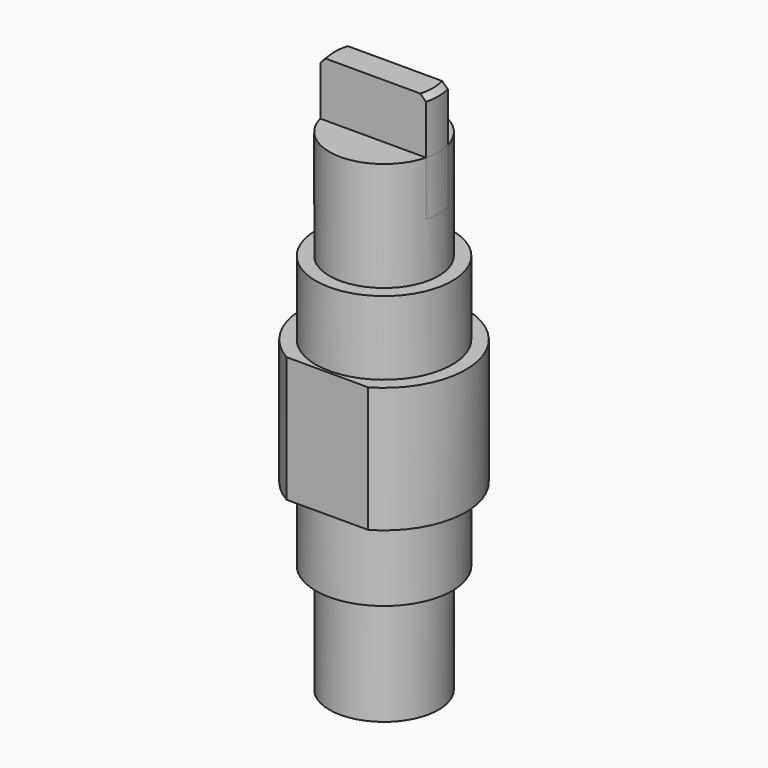
from build123d import *
from build123d import SkipClean  # not in build123d's __all__

# Parameters (mm, degrees)
F3_DEPTH      = 25
F3_DEPTH_BACK = 25
F6_DEPTH      = 10
F6_DEPTH_BACK = 10
F7_SIZE       = 1


with BuildPart() as f1:
    # F0 (on Front) → F1 (revolve)
    with BuildSketch(Plane.XZ):
        Polygon((-12.5, 11.5), (-15, 11.5), (-15, 0), (-15, -11.5), (-12.5, -11.5), (-12.5, -25), (-10, -25), (-10, -45), (0, -45), (0, 0), (0, 45), (-10, 45), (-10, 25), (-12.5, 25), align=None)
    revolve(axis=Axis((0, 0, 22.5), (0, 0, -1)))

    # F2 (on Top) → F3 (cut, two sides)
    with BuildSketch(Plane.XY) as f3_sk:
        Polygon((0, -13), (-15, -13), (-15, -17), (0, -17), (15, -17), (15, -13), align=None)
    extrude(amount=F3_DEPTH, mode=Mode.SUBTRACT)
    extrude(f3_sk.sketch, amount=-F3_DEPTH_BACK, mode=Mode.SUBTRACT)

    # F5 (on offset) → F6 (join, two sides)
    with BuildSketch(Plane.XY.offset(45)) as f6_sk:
        with BuildLine():
            Line((9.6824583655, 2.5), (-9.6824583655, 2.5))
            ThreePointArc((-9.6824583655, 2.5), (-10, 0), (-9.6824583655, -2.5))
            Line((-9.6824583655, -2.5), (9.6824583655, -2.5))
            ThreePointArc((9.6824583655, -2.5), (10, 0), (9.6824583655, 2.5))
        make_face()
    with SkipClean():  # cleaning this boolean's faces spoils the solid; the shape is the same uncleaned
        extrude(amount=F6_DEPTH)
        extrude(f6_sk.sketch, amount=-F6_DEPTH_BACK)

    # F7
    f7_edges = [f1.edges().sort_by_distance(p)[0] for p in [
        (10, 0, 55),
        (-10, 0, 55),
    ]]
    chamfer(f7_edges, length=F7_SIZE)


solid = f1.part
